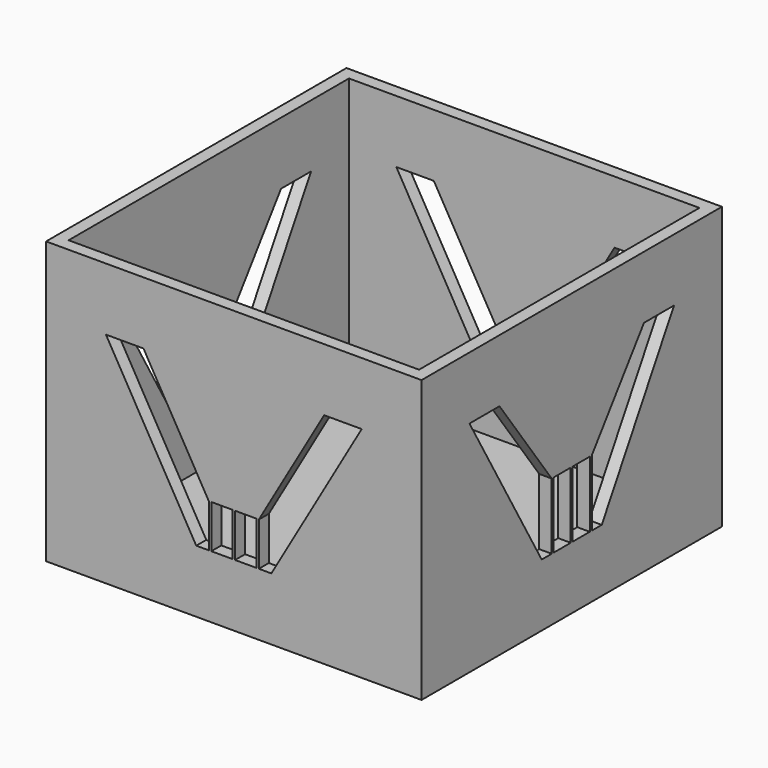
from build123d import *

# Parameters (mm, degrees)
F0_W     = 60
F0_H     = 60
F1_DEPTH = 45
F2_T     = -2
F3_W     = 3.4
F3_H     = 6.9295717942
F4_DEPTH = 64.2
F5_W     = 3.4
F5_H     = 10.5797095255
F6_DEPTH = 63.5
F8_DEPTH = 25


# Not quite as in the source:
# - a feature names something its author has since deleted; it is built from what else it names


with BuildPart() as f1:
    # F0 (on Top) → F1 (new body)
    with BuildSketch(Plane.XY):
        Rectangle(F0_W, F0_H)
    extrude(amount=F1_DEPTH)

    # F2
    f2_openings = [f1.faces().sort_by_distance(p)[0] for p in [
        (0, 0, 45),
    ]]
    offset(amount=F2_T, openings=f2_openings)

    # F3 (on face) → F4 (cut)
    with BuildSketch(Plane.XZ.offset(30)):
        Polygon((-20.4337567297, 35), (-6, 10), (-4, 10), (-4, 16.9295717942), (-14.4337567297, 35), align=None)
        with Locations((-1.9, 13.4647858971)):
            Rectangle(F3_W, F3_H)
        with Locations((1.9, 13.4647858971)):
            Rectangle(F3_W, F3_H)
        Polygon((4, 16.9295717942), (4, 10), (6, 10), (20.4337567297, 35), (14.4337567297, 35), align=None)
    extrude(amount=-F4_DEPTH, mode=Mode.SUBTRACT)

    # F5 (on face) → F6 (cut)
    with BuildSketch(Plane.YZ.offset(30)):
        Polygon((-20.4337567297, 35), (-6, 10), (-4, 10), (-4, 20.5797095255), (-14.4337567297, 35), align=None)
        with Locations((-1.9, 15.2898547627)):
            Rectangle(F5_W, F5_H)
        with Locations((1.9, 15.2898547627)):
            Rectangle(F5_W, F5_H)
        Polygon((4, 20.5797095255), (4, 10), (6, 10), (20.4337567297, 35), (14.4337567297, 35), align=None)
    extrude(amount=-F6_DEPTH, mode=Mode.SUBTRACT)

    # F7 (on face) → F8 (cut)
    with BuildSketch(Plane(origin=(0, 0, 0), x_dir=(1, 0, 0), z_dir=(0, 0, -1))):
        with BuildLine():
            Line((0.9656854249, 0.4), (9.9919967974, 0.4))
            ThreePointArc((9.9919967974, 0.4), (9.2387953251, 3.8268343237), (7.3482514055, 6.7825659806))
            Line((7.3482514055, 6.7825659806), (0.9656854249, 0.4))
        make_face()
        with BuildLine():
            ThreePointArc((7.3482514055, -6.7825659806), (9.2387953251, -3.8268343237), (9.9919967974, -0.4))
            Line((9.9919967974, -0.4), (0.9656854249, -0.4))
            Line((0.9656854249, -0.4), (7.3482514055, -6.7825659806))
        make_face()
        with BuildLine():
            Line((0.4, 0.9656854249), (6.7825659806, 7.3482514055))
            ThreePointArc((6.7825659806, 7.3482514055), (3.8268343237, 9.2387953251), (0.4, 9.9919967974))
            Line((0.4, 9.9919967974), (0.4, 0.9656854249))
        make_face()
        with BuildLine():
            ThreePointArc((0.4, -9.9919967974), (3.8268343237, -9.2387953251), (6.7825659806, -7.3482514055))
            Line((6.7825659806, -7.3482514055), (0.4, -0.9656854249))
            Line((0.4, -0.9656854249), (0.4, -9.9919967974))
        make_face()
        with BuildLine():
            Line((-6.7825659806, 7.3482514055), (-0.4, 0.9656854249))
            Line((-0.4, 0.9656854249), (-0.4, 9.9919967974))
            ThreePointArc((-0.4, 9.9919967974), (-3.8268343237, 9.2387953251), (-6.7825659806, 7.3482514055))
        make_face()
        with BuildLine():
            Line((-0.4, -9.9919967974), (-0.4, -0.9656854249))
            Line((-0.4, -0.9656854249), (-6.7825659806, -7.3482514055))
            ThreePointArc((-6.7825659806, -7.3482514055), (-3.8268343237, -9.2387953251), (-0.4, -9.9919967974))
        make_face()
        with BuildLine():
            Line((-7.3482514055, -6.7825659806), (-0.9656854249, -0.4))
            Line((-0.9656854249, -0.4), (-9.9919967974, -0.4))
            ThreePointArc((-9.9919967974, -0.4), (-9.2387953251, -3.8268343237), (-7.3482514055, -6.7825659806))
        make_face()
        with BuildLine():
            Line((-9.9919967974, 0.4), (-0.9656854249, 0.4))
            Line((-0.9656854249, 0.4), (-7.3482514055, 6.7825659806))
            ThreePointArc((-7.3482514055, 6.7825659806), (-9.2387953251, 3.8268343237), (-9.9919967974, 0.4))
        make_face()
    extrude(amount=-F8_DEPTH, mode=Mode.SUBTRACT)


solid = f1.part
